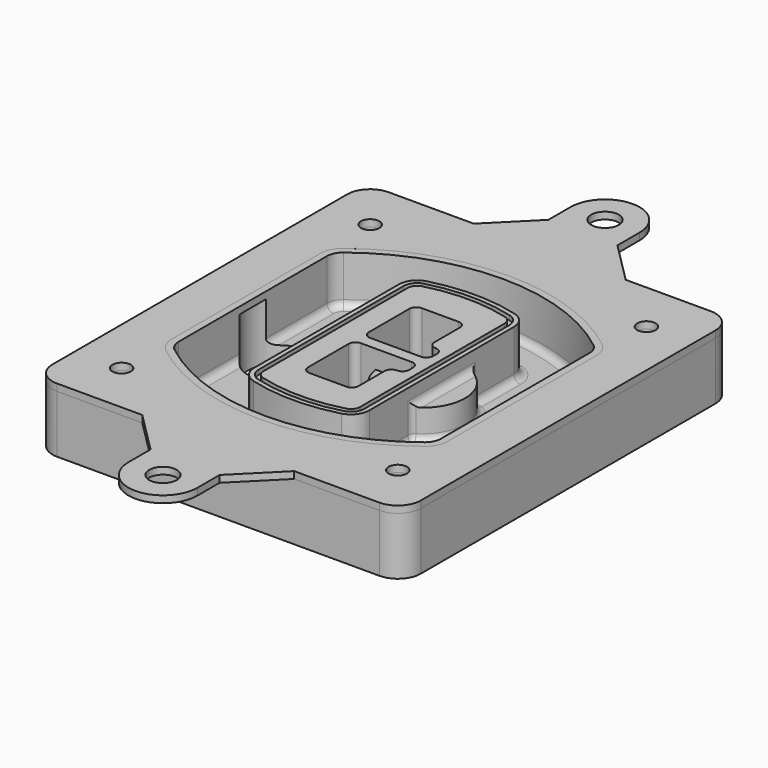
from build123d import *

# Parameters (mm, degrees)
F0_R      = 4
F1_DEPTH  = 25
F2_DEPTH  = 3
F3_DEPTH  = 18
F5_DEPTH  = 21
F6_DEPTH  = 2
F8_DEPTH  = 20
F9_DEPTH  = 16
F10_DEPTH = 25
F7_R      = 6
F7_R_2    = 4
F11_DEPTH = 6
F13_DEPTH = 9
F14_R     = 3
F15_R     = 6
F15_R_2   = 4
F16_DEPTH = 3


# Not quite as in the source:
# - a feature of the source that left no trace in its solid (it failed there, or was rolled back) is left out


with BuildPart() as f1:
    # F0 (on Top) → F1 (new body)
    with BuildSketch(Plane.XY):
        with BuildLine():
            ThreePointArc((-80, -80), (-77.0710678119, -87.0710678119), (-70, -90))
            Line((-70, -90), (70, -90))
            ThreePointArc((70, -90), (77.0710678119, -87.0710678119), (80, -80))
            Line((80, -80), (80, 80))
            ThreePointArc((80, 80), (77.0710678119, 87.0710678119), (70, 90))
            Line((70, 90), (-70, 90))
            ThreePointArc((-70, 90), (-77.0710678119, 87.0710678119), (-80, 80))
            Line((-80, 80), (-80, -80))
        make_face()
        with Locations((-60, -67.5)):
            Circle(F0_R, mode=Mode.SUBTRACT)
        with Locations((60, -67.5)):
            Circle(F0_R, mode=Mode.SUBTRACT)
        with Locations((-60, 67.5)):
            Circle(F0_R, mode=Mode.SUBTRACT)
        with BuildLine():
            ThreePointArc((-64, 40.2934422872), (-62.5820384798, 46.4328484224), (-58.6153846154, 51.3286200352))
            ThreePointArc((-58.6153846154, 51.3286200352), (0, 71.5), (58.6153846154, 51.3286200352))
            ThreePointArc((58.6153846154, 51.3286200352), (62.5820384798, 46.4328484224), (64, 40.2934422872))
            Line((64, 40.2934422872), (64, -40.2934422872))
            ThreePointArc((64, -40.2934422872), (62.5820384798, -46.4328484224), (58.6153846154, -51.3286200352))
            ThreePointArc((58.6153846154, -51.3286200352), (0, -71.5), (-58.6153846154, -51.3286200352))
            ThreePointArc((-58.6153846154, -51.3286200352), (-62.5820384798, -46.4328484224), (-64, -40.2934422872))
            Line((-64, -40.2934422872), (-64, 40.2934422872))
        make_face(mode=Mode.SUBTRACT)
        with Locations((60, 67.5)):
            Circle(F0_R, mode=Mode.SUBTRACT)
        with BuildLine():
            ThreePointArc((58.6153846154, 51.3286200352), (0, 71.5), (-58.6153846154, 51.3286200352))
            ThreePointArc((-58.6153846154, 51.3286200352), (-62.5820384798, 46.4328484224), (-64, 40.2934422872))
            Line((-64, 40.2934422872), (-64, -40.2934422872))
            ThreePointArc((-64, -40.2934422872), (-62.5820384798, -46.4328484224), (-58.6153846154, -51.3286200352))
            ThreePointArc((-58.6153846154, -51.3286200352), (0, -71.5), (58.6153846154, -51.3286200352))
            ThreePointArc((58.6153846154, -51.3286200352), (62.5820384798, -46.4328484224), (64, -40.2934422872))
            Line((64, -40.2934422872), (64, 40.2934422872))
            ThreePointArc((64, 40.2934422872), (62.5820384798, 46.4328484224), (58.6153846154, 51.3286200352))
        make_face()
        with BuildLine():
            Line((-60, -40.2934422872), (-60, 40.2934422872))
            ThreePointArc((-60, 40.2934422872), (-58.9871703427, 44.6787323838), (-56.1538461538, 48.1757121072))
            ThreePointArc((-56.1538461538, 48.1757121072), (0, 67.5), (56.1538461538, 48.1757121072))
            ThreePointArc((56.1538461538, 48.1757121072), (58.9871703427, 44.6787323838), (60, 40.2934422872))
            Line((60, 40.2934422872), (60, -40.2934422872))
            ThreePointArc((60, -40.2934422872), (58.9871703427, -44.6787323838), (56.1538461538, -48.1757121072))
            ThreePointArc((56.1538461538, -48.1757121072), (0, -67.5), (-56.1538461538, -48.1757121072))
            ThreePointArc((-56.1538461538, -48.1757121072), (-58.9871703427, -44.6787323838), (-60, -40.2934422872))
        make_face(mode=Mode.SUBTRACT)
        with BuildLine():
            ThreePointArc((-56.1538461538, 48.1757121072), (-58.9871703427, 44.6787323838), (-60, 40.2934422872))
            Line((-60, 40.2934422872), (-60, -40.2934422872))
            ThreePointArc((-60, -40.2934422872), (-58.9871703427, -44.6787323838), (-56.1538461538, -48.1757121072))
            ThreePointArc((-56.1538461538, -48.1757121072), (0, -67.5), (56.1538461538, -48.1757121072))
            ThreePointArc((56.1538461538, -48.1757121072), (58.9871703427, -44.6787323838), (60, -40.2934422872))
            Line((60, -40.2934422872), (60, 40.2934422872))
            ThreePointArc((60, 40.2934422872), (58.9871703427, 44.6787323838), (56.1538461538, 48.1757121072))
            ThreePointArc((56.1538461538, 48.1757121072), (0, 67.5), (-56.1538461538, 48.1757121072))
        make_face()
        with BuildLine():
            ThreePointArc((54.3076923077, 45.8110311612), (56.2910192399, 43.3631453548), (57, 40.2934422872))
            Line((57, 40.2934422872), (57, -40.2934422872))
            ThreePointArc((57, -40.2934422872), (56.2910192399, -43.3631453548), (54.3076923077, -45.8110311612))
            ThreePointArc((54.3076923077, -45.8110311612), (0, -64.5), (-54.3076923077, -45.8110311612))
            ThreePointArc((-54.3076923077, -45.8110311612), (-56.2910192399, -43.3631453548), (-57, -40.2934422872))
            Line((-57, -40.2934422872), (-57, 40.2934422872))
            ThreePointArc((-57, 40.2934422872), (-56.2910192399, 43.3631453548), (-54.3076923077, 45.8110311612))
            ThreePointArc((-54.3076923077, 45.8110311612), (0, 64.5), (54.3076923077, 45.8110311612))
        make_face(mode=Mode.SUBTRACT)
        with BuildLine():
            Line((57, -40.2934422872), (57, 40.2934422872))
            ThreePointArc((57, 40.2934422872), (56.2910192399, 43.3631453548), (54.3076923077, 45.8110311612))
            ThreePointArc((54.3076923077, 45.8110311612), (0, 64.5), (-54.3076923077, 45.8110311612))
            ThreePointArc((-54.3076923077, 45.8110311612), (-56.2910192399, 43.3631453548), (-57, 40.2934422872))
            Line((-57, 40.2934422872), (-57, -40.2934422872))
            ThreePointArc((-57, -40.2934422872), (-56.2910192399, -43.3631453548), (-54.3076923077, -45.8110311612))
            ThreePointArc((-54.3076923077, -45.8110311612), (0, -64.5), (54.3076923077, -45.8110311612))
            ThreePointArc((54.3076923077, -45.8110311612), (56.2910192399, -43.3631453548), (57, -40.2934422872))
        make_face()
    extrude(amount=-F1_DEPTH)

    # F0 (on Top) → F2 (join)
    with BuildSketch(Plane.XY):
        with BuildLine():
            ThreePointArc((-56.1538461538, 48.1757121072), (-58.9871703427, 44.6787323838), (-60, 40.2934422872))
            Line((-60, 40.2934422872), (-60, -40.2934422872))
            ThreePointArc((-60, -40.2934422872), (-58.9871703427, -44.6787323838), (-56.1538461538, -48.1757121072))
            ThreePointArc((-56.1538461538, -48.1757121072), (0, -67.5), (56.1538461538, -48.1757121072))
            ThreePointArc((56.1538461538, -48.1757121072), (58.9871703427, -44.6787323838), (60, -40.2934422872))
            Line((60, -40.2934422872), (60, 40.2934422872))
            ThreePointArc((60, 40.2934422872), (58.9871703427, 44.6787323838), (56.1538461538, 48.1757121072))
            ThreePointArc((56.1538461538, 48.1757121072), (0, 67.5), (-56.1538461538, 48.1757121072))
        make_face()
        with BuildLine():
            ThreePointArc((54.3076923077, 45.8110311612), (56.2910192399, 43.3631453548), (57, 40.2934422872))
            Line((57, 40.2934422872), (57, -40.2934422872))
            ThreePointArc((57, -40.2934422872), (56.2910192399, -43.3631453548), (54.3076923077, -45.8110311612))
            ThreePointArc((54.3076923077, -45.8110311612), (0, -64.5), (-54.3076923077, -45.8110311612))
            ThreePointArc((-54.3076923077, -45.8110311612), (-56.2910192399, -43.3631453548), (-57, -40.2934422872))
            Line((-57, -40.2934422872), (-57, 40.2934422872))
            ThreePointArc((-57, 40.2934422872), (-56.2910192399, 43.3631453548), (-54.3076923077, 45.8110311612))
            ThreePointArc((-54.3076923077, 45.8110311612), (0, 64.5), (54.3076923077, 45.8110311612))
        make_face(mode=Mode.SUBTRACT)
    extrude(amount=F2_DEPTH)

    # F0 (on Top) → F3 (cut)
    with BuildSketch(Plane.XY):
        with BuildLine():
            Line((57, -40.2934422872), (57, 40.2934422872))
            ThreePointArc((57, 40.2934422872), (56.2910192399, 43.3631453548), (54.3076923077, 45.8110311612))
            ThreePointArc((54.3076923077, 45.8110311612), (0, 64.5), (-54.3076923077, 45.8110311612))
            ThreePointArc((-54.3076923077, 45.8110311612), (-56.2910192399, 43.3631453548), (-57, 40.2934422872))
            Line((-57, 40.2934422872), (-57, -40.2934422872))
            ThreePointArc((-57, -40.2934422872), (-56.2910192399, -43.3631453548), (-54.3076923077, -45.8110311612))
            ThreePointArc((-54.3076923077, -45.8110311612), (0, -64.5), (54.3076923077, -45.8110311612))
            ThreePointArc((54.3076923077, -45.8110311612), (56.2910192399, -43.3631453548), (57, -40.2934422872))
        make_face()
    extrude(amount=-F3_DEPTH, mode=Mode.SUBTRACT)

    # F4 (on face) → F5 (join, through all)
    with BuildSketch(Plane.XY.offset(3)):
        with BuildLine():
            ThreePointArc((-25, -39.2465276821), (-23.3511545998, -44.1109737193), (-19.0842911877, -46.9702398883))
            ThreePointArc((-19.0842911877, -46.9702398883), (0, -49.5), (19.0842911877, -46.9702398883))
            ThreePointArc((19.0842911877, -46.9702398883), (23.3511545998, -44.1109737193), (25, -39.2465276821))
            Line((25, -39.2465276821), (25, 39.2465276821))
            ThreePointArc((25, 39.2465276821), (23.3511545998, 44.1109737193), (19.0842911877, 46.9702398883))
            ThreePointArc((19.0842911877, 46.9702398883), (0, 49.5), (-19.0842911877, 46.9702398883))
            ThreePointArc((-19.0842911877, 46.9702398883), (-23.3511545998, 44.1109737193), (-25, 39.2465276821))
            Line((-25, 39.2465276821), (-25, -39.2465276821))
        make_face()
        with BuildLine():
            ThreePointArc((18.5632183908, 45.0393118368), (21.7633659499, 42.89486221), (23, 39.2465276821))
            Line((23, 39.2465276821), (23, -39.2465276821))
            ThreePointArc((23, -39.2465276821), (21.7633659499, -42.89486221), (18.5632183908, -45.0393118368))
            ThreePointArc((18.5632183908, -45.0393118368), (0, -47.5), (-18.5632183908, -45.0393118368))
            ThreePointArc((-18.5632183908, -45.0393118368), (-21.7633659499, -42.89486221), (-23, -39.2465276821))
            Line((-23, -39.2465276821), (-23, 39.2465276821))
            ThreePointArc((-23, 39.2465276821), (-21.7633659499, 42.89486221), (-18.5632183908, 45.0393118368))
            ThreePointArc((-18.5632183908, 45.0393118368), (0, 47.5), (18.5632183908, 45.0393118368))
        make_face(mode=Mode.SUBTRACT)
        with BuildLine():
            Line((23, -39.2465276821), (23, 39.2465276821))
            ThreePointArc((23, 39.2465276821), (21.7633659499, 42.89486221), (18.5632183908, 45.0393118368))
            ThreePointArc((18.5632183908, 45.0393118368), (0, 47.5), (-18.5632183908, 45.0393118368))
            ThreePointArc((-18.5632183908, 45.0393118368), (-21.7633659499, 42.89486221), (-23, 39.2465276821))
            Line((-23, 39.2465276821), (-23, -39.2465276821))
            ThreePointArc((-23, -39.2465276821), (-21.7633659499, -42.89486221), (-18.5632183908, -45.0393118368))
            ThreePointArc((-18.5632183908, -45.0393118368), (0, -47.5), (18.5632183908, -45.0393118368))
            ThreePointArc((18.5632183908, -45.0393118368), (21.7633659499, -42.89486221), (23, -39.2465276821))
        make_face()
        with BuildLine():
            ThreePointArc((18.0421455939, 43.1083837852), (20.1755772999, 41.6787507007), (21, 39.2465276821))
            Line((21, 39.2465276821), (21, -39.2465276821))
            ThreePointArc((21, -39.2465276821), (20.1755772999, -41.6787507007), (18.0421455939, -43.1083837852))
            ThreePointArc((18.0421455939, -43.1083837852), (0, -45.5), (-18.0421455939, -43.1083837852))
            ThreePointArc((-18.0421455939, -43.1083837852), (-20.1755772999, -41.6787507007), (-21, -39.2465276821))
            Line((-21, -39.2465276821), (-21, 39.2465276821))
            ThreePointArc((-21, 39.2465276821), (-20.1755772999, 41.6787507007), (-18.0421455939, 43.1083837852))
            ThreePointArc((-18.0421455939, 43.1083837852), (0, 45.5), (18.0421455939, 43.1083837852))
        make_face(mode=Mode.SUBTRACT)
        with BuildLine():
            Line((21, -39.2465276821), (21, 39.2465276821))
            ThreePointArc((21, 39.2465276821), (20.1755772999, 41.6787507007), (18.0421455939, 43.1083837852))
            ThreePointArc((18.0421455939, 43.1083837852), (0, 45.5), (-18.0421455939, 43.1083837852))
            ThreePointArc((-18.0421455939, 43.1083837852), (-20.1755772999, 41.6787507007), (-21, 39.2465276821))
            Line((-21, 39.2465276821), (-21, -39.2465276821))
            ThreePointArc((-21, -39.2465276821), (-20.1755772999, -41.6787507007), (-18.0421455939, -43.1083837852))
            ThreePointArc((-18.0421455939, -43.1083837852), (0, -45.5), (18.0421455939, -43.1083837852))
            ThreePointArc((18.0421455939, -43.1083837852), (20.1755772999, -41.6787507007), (21, -39.2465276821))
        make_face()
        with BuildLine():
            Line((-8, -2.5), (14, -2.5))
            ThreePointArc((14, -2.5), (16.1213203436, -3.3786796564), (17, -5.5))
            Line((17, -5.5), (17, -7.5))
            ThreePointArc((17, -7.5), (16.1213203436, -9.6213203436), (14, -10.5))
            ThreePointArc((14, -10.5), (11.8786796564, -11.3786796564), (11, -13.5))
            Line((11, -13.5), (11, -27.5))
            ThreePointArc((11, -27.5), (10.1213203436, -29.6213203436), (8, -30.5))
            Line((8, -30.5), (-8, -30.5))
            ThreePointArc((-8, -30.5), (-10.1213203436, -29.6213203436), (-11, -27.5))
            Line((-11, -27.5), (-11, -5.5))
            ThreePointArc((-11, -5.5), (-10.1213203436, -3.3786796564), (-8, -2.5))
        make_face(mode=Mode.SUBTRACT)
        with BuildLine():
            ThreePointArc((-8, 2.5), (-10.1213203436, 3.3786796564), (-11, 5.5))
            Line((-11, 5.5), (-11, 27.5))
            ThreePointArc((-11, 27.5), (-10.1213203436, 29.6213203436), (-8, 30.5))
            Line((-8, 30.5), (8, 30.5))
            ThreePointArc((8, 30.5), (10.1213203436, 29.6213203436), (11, 27.5))
            Line((11, 27.5), (11, 13.5))
            ThreePointArc((11, 13.5), (11.8786796564, 11.3786796564), (14, 10.5))
            ThreePointArc((14, 10.5), (16.1213203436, 9.6213203436), (17, 7.5))
            Line((17, 7.5), (17, 5.5))
            ThreePointArc((17, 5.5), (16.1213203436, 3.3786796564), (14, 2.5))
            Line((14, 2.5), (-8, 2.5))
        make_face(mode=Mode.SUBTRACT)
    extrude(amount=-F5_DEPTH)

    # F4 (on face) → F6 (cut)
    with BuildSketch(Plane.XY.offset(3)):
        with BuildLine():
            Line((23, -39.2465276821), (23, 39.2465276821))
            ThreePointArc((23, 39.2465276821), (21.7633659499, 42.89486221), (18.5632183908, 45.0393118368))
            ThreePointArc((18.5632183908, 45.0393118368), (0, 47.5), (-18.5632183908, 45.0393118368))
            ThreePointArc((-18.5632183908, 45.0393118368), (-21.7633659499, 42.89486221), (-23, 39.2465276821))
            Line((-23, 39.2465276821), (-23, -39.2465276821))
            ThreePointArc((-23, -39.2465276821), (-21.7633659499, -42.89486221), (-18.5632183908, -45.0393118368))
            ThreePointArc((-18.5632183908, -45.0393118368), (0, -47.5), (18.5632183908, -45.0393118368))
            ThreePointArc((18.5632183908, -45.0393118368), (21.7633659499, -42.89486221), (23, -39.2465276821))
        make_face()
        with BuildLine():
            ThreePointArc((18.0421455939, 43.1083837852), (20.1755772999, 41.6787507007), (21, 39.2465276821))
            Line((21, 39.2465276821), (21, -39.2465276821))
            ThreePointArc((21, -39.2465276821), (20.1755772999, -41.6787507007), (18.0421455939, -43.1083837852))
            ThreePointArc((18.0421455939, -43.1083837852), (0, -45.5), (-18.0421455939, -43.1083837852))
            ThreePointArc((-18.0421455939, -43.1083837852), (-20.1755772999, -41.6787507007), (-21, -39.2465276821))
            Line((-21, -39.2465276821), (-21, 39.2465276821))
            ThreePointArc((-21, 39.2465276821), (-20.1755772999, 41.6787507007), (-18.0421455939, 43.1083837852))
            ThreePointArc((-18.0421455939, 43.1083837852), (0, 45.5), (18.0421455939, 43.1083837852))
        make_face(mode=Mode.SUBTRACT)
    extrude(amount=-F6_DEPTH, mode=Mode.SUBTRACT)

    # F7 (on face) → F8 (join)
    with BuildSketch(Plane(origin=(0, 0, -25), x_dir=(1, 0, 0), z_dir=(0, 0, -1))):
        with BuildLine():
            ThreePointArc((3.28842436, 0), (16.7567035675, 13.4682792075), (30.224982775, 0))
            Line((30.224982775, 0), (35.224982775, 0))
            ThreePointArc((35.224982775, 0), (16.7567035675, 18.4682792075), (-1.71157564, 0))
            Line((-1.71157564, 0), (3.28842436, 0))
        make_face()
        with BuildLine():
            Line((3.28842436, 0), (30.224982775, 0))
            ThreePointArc((30.224982775, 0), (16.7567035675, 13.4682792075), (3.28842436, 0))
        make_face()
        with BuildLine():
            ThreePointArc((3.28842436, 0), (16.7567035675, -13.4682792075), (30.224982775, 0))
            Line((30.224982775, 0), (3.28842436, 0))
        make_face()
        with BuildLine():
            Line((35.224982775, 0), (30.224982775, 0))
            ThreePointArc((30.224982775, 0), (16.7567035675, -13.4682792075), (3.28842436, 0))
            Line((3.28842436, 0), (-1.71157564, 0))
            ThreePointArc((-1.71157564, 0), (16.7567035675, -18.4682792075), (35.224982775, 0))
        make_face()
    extrude(amount=-F8_DEPTH)

    # F7 (on face) → F9 (cut)
    with BuildSketch(Plane(origin=(0, 0, -25), x_dir=(1, 0, 0), z_dir=(0, 0, -1))):
        with BuildLine():
            Line((3.28842436, 0), (30.224982775, 0))
            ThreePointArc((30.224982775, 0), (16.7567035675, 13.4682792075), (3.28842436, 0))
        make_face()
        with BuildLine():
            ThreePointArc((3.28842436, 0), (16.7567035675, -13.4682792075), (30.224982775, 0))
            Line((30.224982775, 0), (3.28842436, 0))
        make_face()
    extrude(amount=-F9_DEPTH, mode=Mode.SUBTRACT)

    # F7 (on face) → F10 (cut)
    with BuildSketch(Plane(origin=(0, 0, -25), x_dir=(1, 0, 0), z_dir=(0, 0, -1))):
        with BuildLine():
            Line((-59.0318229325, 0), (-32.0952645175, 0))
            ThreePointArc((-32.0952645175, 0), (-45.563543725, 13.4682792075), (-59.0318229325, 0))
        make_face()
        with BuildLine():
            ThreePointArc((-59.0318229325, 0), (-45.563543725, -13.4682792075), (-32.0952645175, 0))
            Line((-32.0952645175, 0), (-59.0318229325, 0))
        make_face()
    extrude(amount=-F10_DEPTH, mode=Mode.SUBTRACT)

    # F7 (on face) → F11 (cut)
    with BuildSketch(Plane(origin=(0, 0, -25), x_dir=(1, 0, 0), z_dir=(0, 0, -1))):
        with Locations((60, -67.5)):
            Circle(F7_R)
        with Locations((60, -67.5)):
            Circle(F7_R_2, mode=Mode.SUBTRACT)
        with Locations((-60, -67.5)):
            Circle(F7_R)
        with Locations((-60, -67.5)):
            Circle(F7_R_2, mode=Mode.SUBTRACT)
        with Locations((-60, 67.5)):
            Circle(F7_R)
        with Locations((-60, 67.5)):
            Circle(F7_R_2, mode=Mode.SUBTRACT)
        with Locations((60, 67.5)):
            Circle(F7_R)
        with Locations((60, 67.5)):
            Circle(F7_R_2, mode=Mode.SUBTRACT)
    extrude(amount=-F11_DEPTH, mode=Mode.SUBTRACT)

    # F12 (on face) → F13 (cut, through all)
    with BuildSketch(Plane(origin=(0, 0, -9), x_dir=(1, 0, 0), z_dir=(0, 0, -1))):
        with BuildLine():
            Line((11, 13.5), (11, 17.5481537753))
            ThreePointArc((11, 17.5481537753), (2.5696536419, 11.8239143813), (-1.5415842455, 2.5))
            Line((-1.5415842455, 2.5), (3.5224848595, 2.5))
            ThreePointArc((3.5224848595, 2.5), (6.1857188154, 8.3455872281), (11.2536447004, 12.2927168648))
            ThreePointArc((11.2536447004, 12.2927168648), (11.0640958889, 12.8831798879), (11, 13.5))
        make_face()
        with BuildLine():
            ThreePointArc((11.2536447004, -12.2927168648), (6.1857188154, -8.3455872281), (3.5224848595, -2.5))
            Line((3.5224848595, -2.5), (-1.5415842455, -2.5))
            ThreePointArc((-1.5415842455, -2.5), (2.5696536419, -11.8239143813), (11, -17.5481537753))
            Line((11, -17.5481537753), (11, -13.5))
            ThreePointArc((11, -13.5), (11.0640958889, -12.8831798879), (11.2536447004, -12.2927168648))
        make_face()
        with BuildLine():
            ThreePointArc((11.2536447004, 12.2927168648), (6.1857188154, 8.3455872281), (3.5224848595, 2.5))
            Line((3.5224848595, 2.5), (14, 2.5))
            ThreePointArc((14, 2.5), (16.1213203436, 3.3786796564), (17, 5.5))
            Line((17, 5.5), (17, 7.5))
            ThreePointArc((17, 7.5), (16.1213203436, 9.6213203436), (14, 10.5))
            ThreePointArc((14, 10.5), (12.3601599782, 10.9878446101), (11.2536447004, 12.2927168648))
        make_face()
        with BuildLine():
            Line((14, -2.5), (3.5224848595, -2.5))
            ThreePointArc((3.5224848595, -2.5), (6.1857188154, -8.3455872281), (11.2536447004, -12.2927168648))
            ThreePointArc((11.2536447004, -12.2927168648), (12.3601599782, -10.9878446101), (14, -10.5))
            ThreePointArc((14, -10.5), (16.1213203436, -9.6213203436), (17, -7.5))
            Line((17, -7.5), (17, -5.5))
            ThreePointArc((17, -5.5), (16.1213203436, -3.3786796564), (14, -2.5))
        make_face()
    extrude(amount=F13_DEPTH, mode=Mode.SUBTRACT)

    # F14
    f14_edges = [f1.edges().sort_by_distance(p)[0] for p in [
        (-57, -23.703476, -18),
        (-57, 23.703476, -18),
        (25, 0, -5),
        (25, 16.526506, -11.5),
        (25, -16.526506, -11.5),
        (25, -27.886517, -18),
        (35.224983, 0, -18),
        (23.351155, -44.110974, -18),
        (56.291019, -43.363145, -18),
        (0, -64.5, -18),
        (-56.291019, -43.363145, -18),
        (-56.291019, 43.363145, -18),
        (0, 64.5, -18),
        (56.291019, 43.363145, -18),
        (57, 0, -18),
        (-23.351155, 44.110974, -18),
        (0, 49.5, -18),
        (-25, 0, -18),
        (23.351155, 44.110974, -18),
        (-23.351155, -44.110974, -18),
        (25, 27.886517, -18),
        (0, -49.5, -18),
    ]]
    fillet(f14_edges, radius=F14_R)


with BuildPart() as f16:
    # F15 (on face) → F16 (new body, through all)
    with BuildSketch(Plane.XY):
        with BuildLine():
            Line((15, 108), (15, 120))
            ThreePointArc((15, 120), (0, 135), (-15, 120))
            Line((-15, 120), (-15, 108))
            Line((-15, 108), (-33, 90))
            Line((-33, 90), (33, 90))
            Line((33, 90), (15, 108))
        make_face()
        with Locations((0, 120)):
            Circle(F15_R, mode=Mode.SUBTRACT)
        with BuildLine():
            Line((70, 90), (33, 90))
            Line((33, 90), (-33, 90))
            Line((-33, 90), (-70, 90))
            ThreePointArc((-70, 90), (-77.0710678119, 87.0710678119), (-80, 80))
            Line((-80, 80), (-80, -80))
            ThreePointArc((-80, -80), (-77.0710678119, -87.0710678119), (-70, -90))
            Line((-70, -90), (-33, -90))
            Line((-33, -90), (33, -90))
            Line((33, -90), (70, -90))
            ThreePointArc((70, -90), (77.0710678119, -87.0710678119), (80, -80))
            Line((80, -80), (80, 80))
            ThreePointArc((80, 80), (77.0710678119, 87.0710678119), (70, 90))
        make_face()
        with Locations((-60, -67.5)):
            Circle(F15_R_2, mode=Mode.SUBTRACT)
        with Locations((60, -67.5)):
            Circle(F15_R_2, mode=Mode.SUBTRACT)
        with Locations((-60, 67.5)):
            Circle(F15_R_2, mode=Mode.SUBTRACT)
        with BuildLine():
            ThreePointArc((-60, 40.2934422872), (-58.9871703427, 44.6787323838), (-56.1538461538, 48.1757121072))
            ThreePointArc((-56.1538461538, 48.1757121072), (0, 67.5), (56.1538461538, 48.1757121072))
            ThreePointArc((56.1538461538, 48.1757121072), (58.9871703427, 44.6787323838), (60, 40.2934422872))
            Line((60, 40.2934422872), (60, -40.2934422872))
            ThreePointArc((60, -40.2934422872), (58.9871703427, -44.6787323838), (56.1538461538, -48.1757121072))
            ThreePointArc((56.1538461538, -48.1757121072), (0, -67.5), (-56.1538461538, -48.1757121072))
            ThreePointArc((-56.1538461538, -48.1757121072), (-58.9871703427, -44.6787323838), (-60, -40.2934422872))
            Line((-60, -40.2934422872), (-60, 40.2934422872))
        make_face(mode=Mode.SUBTRACT)
        with Locations((60, 67.5)):
            Circle(F15_R_2, mode=Mode.SUBTRACT)
        with BuildLine():
            Line((15, -108), (33, -90))
            Line((33, -90), (-33, -90))
            Line((-33, -90), (-15, -108))
            Line((-15, -108), (-15, -120))
            ThreePointArc((-15, -120), (0, -135), (15, -120))
            Line((15, -120), (15, -108))
        make_face()
        with Locations((0, -120)):
            Circle(F15_R, mode=Mode.SUBTRACT)
    extrude(amount=F16_DEPTH)


solid = Compound([f1.part, f16.part])
